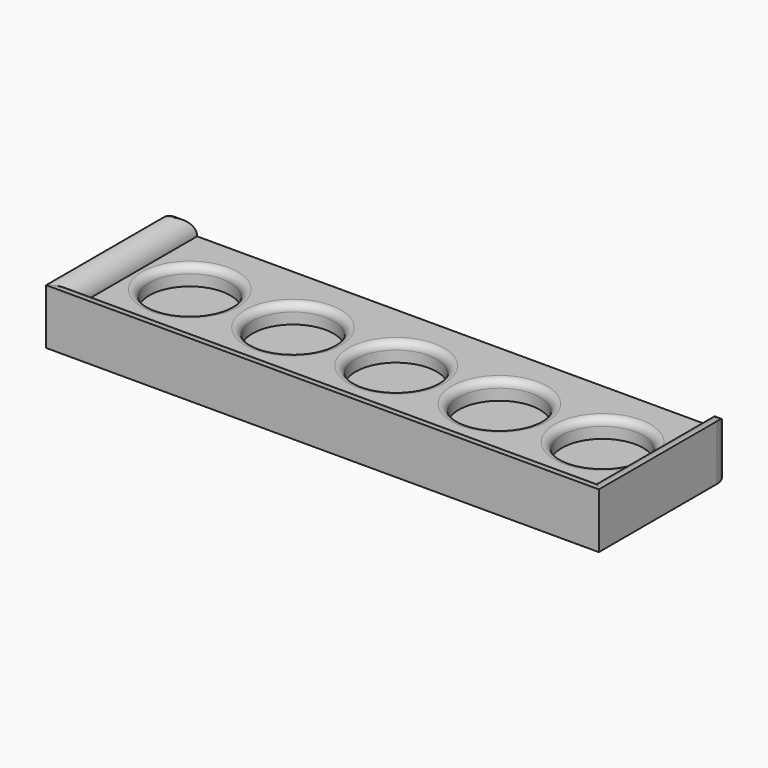
from build123d import *

# Parameters (mm, degrees)
F1_W          = 70
F1_H          = 20
F2_DEPTH      = 2.5
F2_DEPTH_BACK = 2.5
F0_R          = 5.5
F3_DEPTH      = 25.4
F5_DEPTH      = 7.5
F6_R          = 2.49999
F7_R          = 1


# Not quite as in the source:
# - a fillet or chamfer is up to 0.001 mm smaller than in the source, because OpenCascade refuses the exact size


with BuildPart() as f2:
    # F1 (on face) → F2 (new body, two sides)
    with BuildSketch(Plane.XY) as f2_sk:
        with Locations((-180.2211654186, 20.1380707997)):
            Rectangle(F1_W, F1_H)
    extrude(amount=F2_DEPTH)
    extrude(f2_sk.sketch, amount=-F2_DEPTH_BACK)

    # F0 (on Top) → F3 (cut)
    with BuildSketch(Plane.XY):
        with Locations((-152.2211654186, 20.1380707997)):
            Circle(F0_R)
        with Locations((-166.2211654186, 20.1380707997)):
            Circle(F0_R)
        with Locations((-180.2211654186, 20.1380707997)):
            Circle(F0_R)
        with Locations((-194.2211654186, 20.1380707997)):
            Circle(F0_R)
        with Locations((-208.2211654186, 20.1380707997)):
            Circle(F0_R)
    extrude(amount=F3_DEPTH, mode=Mode.SUBTRACT)

    # F7
    f7_edges = [f2.edges().sort_by_distance(p)[0] for p in [
        (-157.721165, 20.138071, 2.5),
        (-171.721165, 20.138071, 2.5),
        (-185.721165, 20.138071, 2.5),
        (-199.721165, 20.138071, 2.5),
        (-213.721165, 20.138071, 2.5),
    ]]
    fillet(f7_edges, radius=F7_R)


with BuildPart() as f5:
    # F4 (on face) → F5 (new body)
    with BuildSketch(Plane(origin=(0, 0, -2.5), x_dir=(1, 0, 0), z_dir=(0, 0, -1))):
        Polygon((-145.2211654186, -30.1380707997), (-142.7211654186, -30.1380707997), (-142.7211654186, -7.6380707997), (-217.7211654186, -7.6380707997), (-217.7211654186, -30.1380707997), (-215.2211654186, -30.1380707997), (-215.2211654186, -10.1380707997), (-145.2211654186, -10.1380707997), align=None)
    extrude(amount=-F5_DEPTH)

    # F6 (radius 2.5 in the source; OpenCascade refuses exactly that, so slightly less here)
    f6_edges = [f5.edges().sort_by_distance(p)[0] for p in [
        (-180.221165, 10.138071, 5),
        (-145.221165, 20.138071, 5),
        (-215.221165, 20.138071, 5),
        (-216.471165, 30.138071, 5),
        (-143.971165, 30.138071, 5),
        (-142.721165, 30.138071, 1.25),
        (-217.721165, 30.138071, 1.25),
    ]]
    fillet(f6_edges, radius=F6_R)


solid = Compound([f2.part, f5.part])
